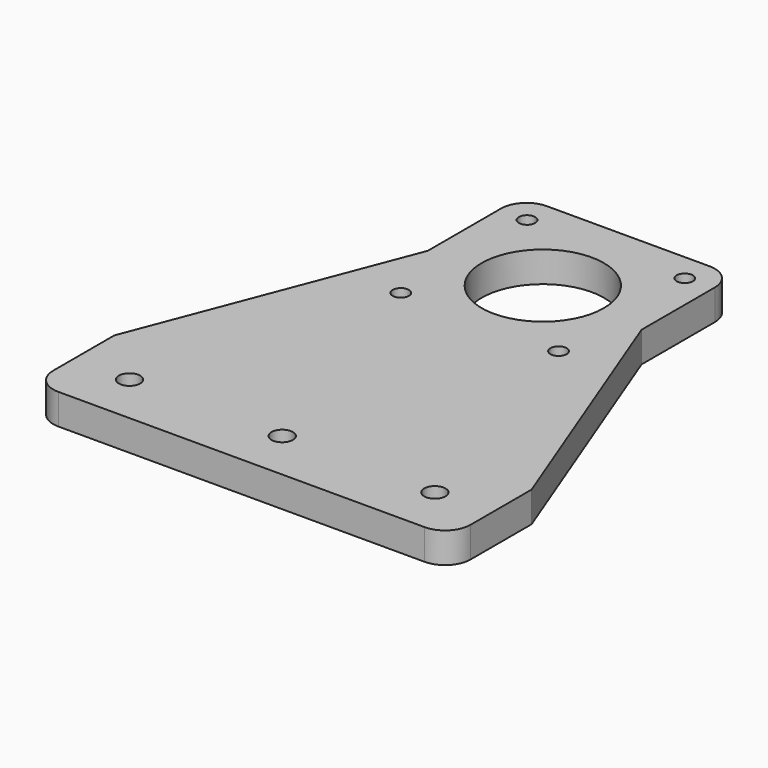
from build123d import *

# Parameters (mm, degrees)
F0_W     = 82
F0_H     = 95
F1_DEPTH = 6
F3_DEPTH = 6.001
F4_R     = 12
F4_R_2   = 1.6
F4_R_3   = 2.1
F5_DEPTH = 6.001
F6_R     = 5


# Not quite as in the source:
# - a pattern or mirror of a feature is missing from the dataset's text; its kind, count and spacing are read off the source's solid


with BuildPart() as f1:
    # F0 (on Top) → F1 (new body)
    with BuildSketch(Plane.XY):
        Rectangle(F0_W, F0_H)
    extrude(amount=F1_DEPTH)

    # F2 (on face) → F3 (cut, through all)
    with BuildSketch(Plane.XY.offset(6)):
        Polygon((-41, -27.5), (-21, 24.5), (-21, 47.5), (-41, 47.5), align=None)
    f3 = extrude(amount=-F3_DEPTH, mode=Mode.SUBTRACT)

    # F3_copies: F3 across plane
    add(f3.mirror(Plane(origin=(0, 0, 0), x_dir=(0, 0, 1), z_dir=(1, 0, 0))), mode=Mode.SUBTRACT)

    # F4 (on face) → F5 (cut, through all)
    with BuildSketch(Plane.XY.offset(6)):
        with Locations((0, 26.5003114)):
            Circle(F4_R)
        with Locations((15.5, 42.0003114)):
            Circle(F4_R_2)
        with Locations((-15.5, 42.0003114)):
            Circle(F4_R_2)
        with Locations((15.5, 11.0003114)):
            Circle(F4_R_2)
        with Locations((-15.5, 11.0003114)):
            Circle(F4_R_2)
        with Locations((-30, -37.5003114)):
            Circle(F4_R_3)
        with Locations((0, -37.5003114)):
            Circle(F4_R_3)
        with Locations((30, -37.5003114)):
            Circle(F4_R_3)
    extrude(amount=-F5_DEPTH, mode=Mode.SUBTRACT)

    # F6
    f6_edges = [f1.edges().sort_by_distance(p)[0] for p in [
        (-41, -47.5, 3),
        (41, -47.5, 3),
        (-21, 47.5, 3),
        (21, 47.5, 3),
    ]]
    fillet(f6_edges, radius=F6_R)


solid = f1.part
